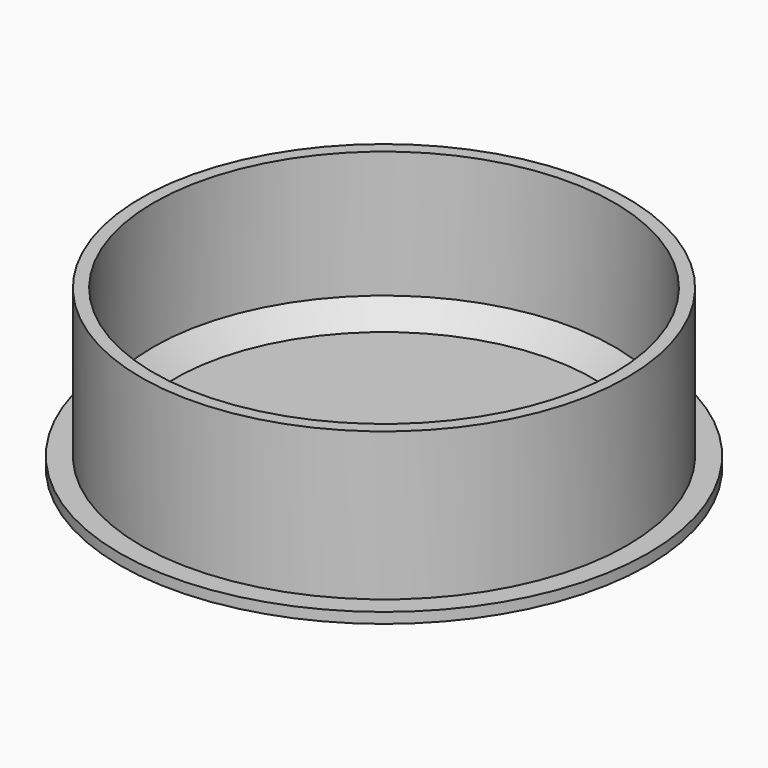
from build123d import *

# Parameters (mm, degrees)
F0_R     = 50
F0_R_2   = 46
F0_R_3   = 43.6
F1_DEPTH = 2
F2_DEPTH = 30
F3_SIZE  = 4


with BuildPart() as f1:
    # F0 (on Top) → F1 (new body)
    with BuildSketch(Plane.XY):
        Circle(F0_R)
        Circle(F0_R_2, mode=Mode.SUBTRACT)
        Circle(F0_R_2)
        Circle(F0_R_3, mode=Mode.SUBTRACT)
        Circle(F0_R_3)
    extrude(amount=F1_DEPTH)

    # F0 (on Top) → F2 (join)
    with BuildSketch(Plane.XY):
        Circle(F0_R_2)
        Circle(F0_R_3, mode=Mode.SUBTRACT)
    extrude(amount=F2_DEPTH)

    # F3
    f3_edges = [f1.edges().sort_by_distance(p)[0] for p in [
        (-43.6, 0, 2),
    ]]
    chamfer(f3_edges, length=F3_SIZE)


solid = f1.part
